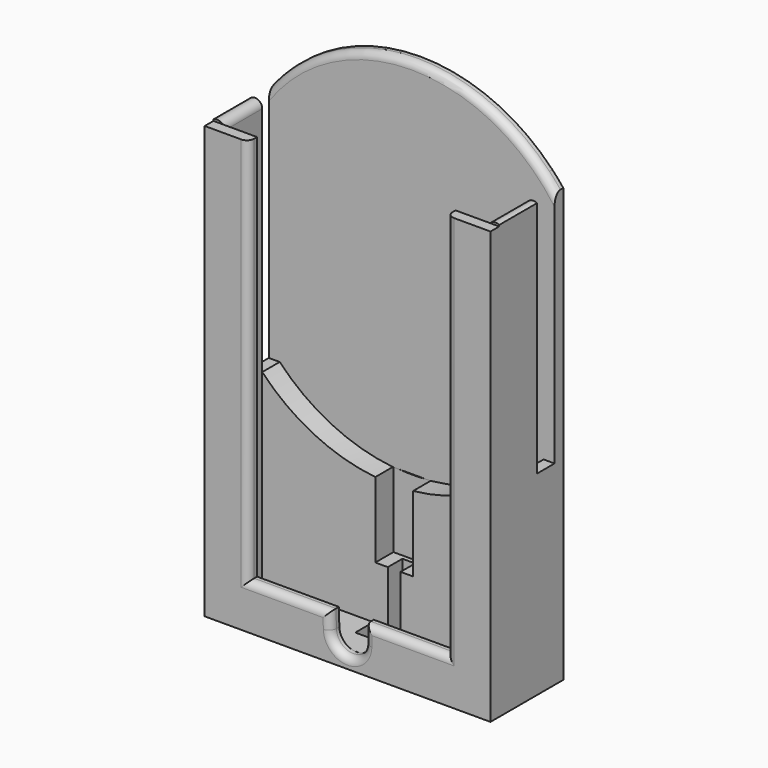
from build123d import *

# Parameters (mm, degrees)
F1_DEPTH      = 3
F2_DEPTH      = 9
F3_DEPTH      = 22
F4_DEPTH      = 22
F5_DEPTH      = 22
F6_W          = 6
F6_H          = 68.8748865698
F7_DEPTH      = 4
F8_W          = 6
F8_H          = 68.8748865698
F9_DEPTH      = 4
F10_DEPTH     = 2.8
F11_W         = 3.5
F11_H         = 14.5974665339
F12_DEPTH     = 5
F14_DEPTH     = 4
F15_DEPTH     = 4
F16_W         = 54.5
F16_H         = 12.2903782427
F17_DEPTH     = 3
F19_DEPTH     = 3
F20_T1_DEPTH  = 111.3131168485
F20_T3_DEPTH  = 27.4743105508
F20_T5_DEPTH  = 27.4558316657
F20_T7_DEPTH  = 9.7989282925
F20_T9_DEPTH  = 13
F20_T11_DEPTH = 9.7709294909
F20_T14_ANGLE = 114.906593859
F20_T16_ANGLE = 177.2719132967
F20_T21_DEPTH = 111.3131168485
F20_T25_DEPTH = 32.4558316657
F20_T32_DEPTH = 32.4743105508
F20_T36_DEPTH = 111.3131168485


# Not quite as in the source:
# - a fillet or chamfer that OpenCascade refuses, or shapes differently, is made with other operations: its cross-section is extruded or revolved along the edge and cut away or added


with BuildPart() as f1:
    # F0 (on Front) → F1 (new body)
    with BuildSketch(Plane.XZ):
        with BuildLine():
            Line((36.25, -19.4374432849), (36.25, 49.4374432849))
            ThreePointArc((36.25, 49.4374432849), (0, 65), (-36.25, 49.4374432849))
            Line((-36.25, 49.4374432849), (-36.25, -19.4374432849))
            ThreePointArc((-36.25, -19.4374432849), (-22.0820535862, -29.8595910527), (-5.1816573471, -34.7307794745))
            Line((-5.1816573471, -34.7307794745), (5.1816573471, -34.7307794745))
            ThreePointArc((5.1816573471, -34.7307794745), (22.0820535862, -29.8595910527), (36.25, -19.4374432849))
        make_face()
    extrude(amount=F1_DEPTH)

    # F0 (on Front) → F2 (join)
    with BuildSketch(Plane.XZ):
        with BuildLine():
            Line((36.25, -70), (36.25, -19.4374432849))
            ThreePointArc((36.25, -19.4374432849), (22.0820535862, -29.8595910527), (5.1816573471, -34.7307794745))
            Line((5.1816573471, -34.7307794745), (5.1816573471, -55.4025334661))
            Line((5.1816573471, -55.4025334661), (-5.1816573471, -55.4025334661))
            Line((-5.1816573471, -55.4025334661), (-5.1816573471, -34.7307794745))
            ThreePointArc((-5.1816573471, -34.7307794745), (-22.0820535862, -29.8595910527), (-36.25, -19.4374432849))
            Line((-36.25, -19.4374432849), (-36.25, -70))
            Line((-36.25, -70), (36.25, -70))
        make_face()
    extrude(amount=F2_DEPTH)

    # F0 (on Front) → F3 (join)
    with BuildSketch(Plane.XZ):
        with BuildLine():
            ThreePointArc((39.25, -15.9747881349), (37.7896810673, -17.7404948776), (36.25, -19.4374432849))
            Line((36.25, -19.4374432849), (36.25, -70))
            Line((36.25, -70), (-36.25, -70))
            Line((-36.25, -70), (-36.25, -19.4374432849))
            ThreePointArc((-36.25, -19.4374432849), (-37.7896810674, -17.7404948776), (-39.25, -15.9747881349))
            Line((-39.25, -15.9747881349), (-39.25, -73))
            Line((-39.25, -73), (39.25, -73))
            Line((39.25, -73), (39.25, -15.9747881349))
        make_face()
    extrude(amount=F3_DEPTH)

    # F0 (on Front) → F4 (join)
    with BuildSketch(Plane.XZ):
        with BuildLine():
            Line((-36.25, -19.4374432849), (-36.25, 49.4374432849))
            ThreePointArc((-36.25, 49.4374432849), (-37.7896810673, 47.7404948776), (-39.25, 45.9747881349))
            Line((-39.25, 45.9747881349), (-39.25, -15.9747881349))
            ThreePointArc((-39.25, -15.9747881349), (-37.7896810674, -17.7404948776), (-36.25, -19.4374432849))
        make_face()
    extrude(amount=F4_DEPTH)

    # F0 (on Front) → F5 (join)
    with BuildSketch(Plane.XZ):
        with BuildLine():
            ThreePointArc((39.25, 45.9747881349), (37.7896810673, 47.7404948776), (36.25, 49.4374432849))
            Line((36.25, 49.4374432849), (36.25, -19.4374432849))
            ThreePointArc((36.25, -19.4374432849), (37.7896810673, -17.7404948776), (39.25, -15.9747881349))
            Line((39.25, -15.9747881349), (39.25, 45.9747881349))
        make_face()
    extrude(amount=F5_DEPTH)

    # F6 (on face) → F7 (cut)
    with BuildSketch(Plane.YZ.offset(-36.25)):
        with Locations((-6, 15)):
            Rectangle(F6_W, F6_H)
    extrude(amount=-F7_DEPTH, mode=Mode.SUBTRACT)

    # F8 (on face) → F9 (cut)
    with BuildSketch(Plane(origin=(36.25, 0, 0), x_dir=(0, -1, 0), z_dir=(-1, 0, 0))):
        with Locations((6, 15)):
            Rectangle(F8_W, F8_H)
    extrude(amount=-F9_DEPTH, mode=Mode.SUBTRACT)

    # F0 (on Front) → F10 (join)
    with BuildSketch(Plane.XZ):
        with BuildLine():
            Line((5.1816573471, -55.4025334661), (5.1816573471, -34.7307794745))
            ThreePointArc((5.1816573471, -34.7307794745), (2.5943232525, -34.9326495077), (0, -35))
            ThreePointArc((0, -35), (-2.5943232525, -34.9326495077), (-5.1816573471, -34.7307794745))
            Line((-5.1816573471, -34.7307794745), (-5.1816573471, -55.4025334661))
            Line((-5.1816573471, -55.4025334661), (5.1816573471, -55.4025334661))
        make_face()
    extrude(amount=F10_DEPTH)

    # F11 (on face) → F12 (cut)
    with BuildSketch(Plane.XZ.offset(9)):
        with Locations((0, -62.7012667331)):
            Rectangle(F11_W, F11_H)
    extrude(amount=-F12_DEPTH, mode=Mode.SUBTRACT)

    # F13 (on face) → F14 (cut)
    with BuildSketch(Plane.XY.offset(-70)):
        Polygon((-1.75, -9), (-5.7336706668, -9), (-5.7336706668, -15.2), (5.8953360592, -15.2), (5.8953360592, -9), (1.75, -9), align=None)
    extrude(amount=-F14_DEPTH, mode=Mode.SUBTRACT)

    # F15 (cut): a face of the model
    f15_faces = [f1.faces().sort_by_distance(p)[0] for p in [
        (0, -6.5, -70),
    ]]
    extrude(f15_faces, amount=-F15_DEPTH, mode=Mode.SUBTRACT)

    # F16 (on face) → F17 (join)
    with BuildSketch(Plane.XZ.offset(22)):
        Polygon((-39.25, 45.6034950912), (-39.25, -73), (-27.25, -73), (-27.25, -60.7096217573), (-27.25, 45.6034950912), align=None)
        with Locations((0, -66.8548108786)):
            Rectangle(F16_W, F16_H)
        Polygon((27.25, -60.7096217573), (27.25, -73), (39.25, -73), (39.25, 45.6034950912), (27.25, 45.6034950912), align=None)
    extrude(amount=F17_DEPTH)

    # F18 (on face) → F19 (cut)
    with BuildSketch(Plane.XZ.offset(25)):
        with BuildLine():
            ThreePointArc((0.0047599162, -60.7096217573), (-3.3429375433, -62.1225677813), (-4.6658988973, -65.5068355016))
            ThreePointArc((-4.6658988973, -65.5068355016), (0.0184260463, -70.0542581163), (4.6760694509, -65.4795110707))
            ThreePointArc((4.6760694509, -65.4795110707), (4.6768334539, -65.4307331593), (4.6770881308, -65.3819499298))
            ThreePointArc((4.6770881308, -65.3819499298), (3.3085948781, -62.0781149802), (0.0047599162, -60.7096217573))
        make_face()
        with BuildLine():
            ThreePointArc((4.6770881308, -65.3819499298), (4.6768334539, -65.4307331593), (4.6760694509, -65.4795110707))
            Line((4.6760694509, -65.4795110707), (4.7756894492, -60.7096217573))
            Line((4.7756894492, -60.7096217573), (0.0047599162, -60.7096217573))
            ThreePointArc((0.0047599162, -60.7096217573), (3.3085948781, -62.0781149802), (4.6770881308, -65.3819499298))
        make_face()
        with BuildLine():
            Line((-4.7941683343, -60.7096217573), (-4.6658988973, -65.5068355016))
            ThreePointArc((-4.6658988973, -65.5068355016), (-3.3429375433, -62.1225677813), (0.0047599162, -60.7096217573))
            Line((0.0047599162, -60.7096217573), (-4.7941683343, -60.7096217573))
        make_face()
    extrude(amount=-F19_DEPTH, mode=Mode.SUBTRACT)

    # F20: fillet of radius 2 on 10 edges, made by hand

    # F20_s2 → F20_t1 (cut)
    with BuildSketch(Plane.XY.offset(-60.7096217573)):
        with BuildLine():
            ThreePointArc((-29.25, -25), (-27.8357864376, -24.4142135624), (-27.25, -23))
            Line((-27.25, -23), (-27.25, -25))
            Line((-27.25, -25), (-29.25, -25))
        make_face()
        with BuildLine():
            ThreePointArc((29.25, -25), (27.8357864376, -24.4142135624), (27.25, -23))
            Line((27.25, -23), (27.25, -25))
            Line((27.25, -25), (29.25, -25))
        make_face()
    extrude(amount=F20_T1_DEPTH, mode=Mode.SUBTRACT)

    # F20_s4 → F20_t3 (cut)
    with BuildSketch(Plane.YZ.offset(-0.2243105508)):
        with BuildLine():
            ThreePointArc((-25, -62.7096217573), (-24.4142135624, -61.2954081949), (-23, -60.7096217573))
            Line((-23, -60.7096217573), (-25, -60.7096217573))
            Line((-25, -60.7096217573), (-25, -62.7096217573))
        make_face()
    extrude(amount=F20_T3_DEPTH, mode=Mode.SUBTRACT)

    # F20_s6 → F20_t5 (cut)
    with BuildSketch(Plane.YZ.offset(-27.25)):
        with BuildLine():
            ThreePointArc((-25, -62.7096217573), (-24.4142135624, -61.2954081949), (-23, -60.7096217573))
            Line((-23, -60.7096217573), (-25, -60.7096217573))
            Line((-25, -60.7096217573), (-25, -62.7096217573))
        make_face()
    extrude(amount=F20_T5_DEPTH, mode=Mode.SUBTRACT)

    # F20_s8 → F20_t7 (cut)
    with BuildSketch(Plane(origin=(1.4850446734, 0, -55.5399391245), x_dir=(0, 1, 0), z_dir=(0.0267287672, 0, -0.9996427227))):
        with BuildLine():
            ThreePointArc((-25, -8.4151488306), (-24.4142135624, -7.0009352682), (-23, -6.4151488306))
            Line((-23, -6.4151488306), (-25, -6.4151488306))
            Line((-25, -6.4151488306), (-25, -8.4151488306))
        make_face()
    extrude(amount=F20_T7_DEPTH, mode=Mode.SUBTRACT)

    # F20_s10 → F20_t9 (cut)
    with BuildSketch(Plane.XZ.offset(9)):
        with BuildLine():
            ThreePointArc((39.25, 45.9747881349), (37.25, 45.9747881349), (36.25, 44.2427373273))
            Line((36.25, 44.2427373273), (36.25, 49.4374432849))
            ThreePointArc((36.25, 49.4374432849), (37.7896810673, 47.7404948776), (39.25, 45.9747881349))
        make_face()
        with BuildLine():
            ThreePointArc((-39.25, 45.9747881349), (-37.25, 45.9747881349), (-36.25, 44.2427373273))
            Line((-36.25, 44.2427373273), (-36.25, 49.4374432849))
            ThreePointArc((-36.25, 49.4374432849), (-37.7896810673, 47.7404948776), (-39.25, 45.9747881349))
        make_face()
    extrude(amount=F20_T9_DEPTH, mode=Mode.SUBTRACT)

    # F20_s12 → F20_t11 (cut)
    with BuildSketch(Plane(origin=(-1.3649163722, 0, -65.3533439927), x_dir=(0, 1, 0), z_dir=(0.0208806268, 0, 0.9997819759))):
        with BuildLine():
            ThreePointArc((-25, -8.0423031905), (-24.4142135624, -6.6280896281), (-23, -6.0423031905))
            Line((-23, -6.0423031905), (-25, -6.0423031905))
            Line((-25, -6.0423031905), (-25, -8.0423031905))
        make_face()
    extrude(amount=F20_T11_DEPTH, mode=Mode.SUBTRACT)

    # F20_s13 → F20_t14 (revolve, cut)
    with BuildSketch(Plane(origin=(6.8024666518, 0, 10.65855148), x_dir=(0, 1, 0), z_dir=(-0.537986897, 0, -0.8429532008))):
        with BuildLine():
            ThreePointArc((-1, -58.0698034549), (-2.4142135624, -57.4840170172), (-3, -56.0698034549))
            Line((-3, -56.0698034549), (-3, -58.0698034549))
            Line((-3, -58.0698034549), (-1, -58.0698034549))
        make_face()
    revolve(axis=Axis((0, -3, 15), (0, 1, 0)), revolution_arc=F20_T14_ANGLE, mode=Mode.SUBTRACT)

    # F20_s15 → F20_t16 (revolve, cut)
    with BuildSketch(Plane(origin=(1.746957946, 0, -65.3353664822), x_dir=(0, 1, 0), z_dir=(-0.0267287672, 0, 0.9996427227))):
        with BuildLine():
            ThreePointArc((-25, 8.4151488306), (-24.4142135624, 7.0009352682), (-23, 6.4151488306))
            Line((-23, 6.4151488306), (-25, 6.4151488306))
            Line((-25, 6.4151488306), (-25, 8.4151488306))
        make_face()
    revolve(axis=Axis((0.0047599583, -25, -65.3819499298), (0, -1, 0)), revolution_arc=F20_T16_ANGLE, mode=Mode.SUBTRACT)


with BuildPart() as f20_tool19:
    # F20_s20 → F20_t21 (new body)
    with BuildSketch(Plane.XY.offset(-65.7096217573)):
        with BuildLine():
            ThreePointArc((-29.25, -25), (-27.8357864376, -24.4142135624), (-27.25, -23))
            Line((-27.25, -23), (-27.25, -25))
            Line((-27.25, -25), (-29.25, -25))
        make_face()
    extrude(amount=F20_T21_DEPTH)

    split(bisect_by=Plane.XY.offset(-60.7096217573), keep=Keep.BOTTOM)


with BuildPart() as f20_tool23:
    # F20_s24 → F20_t25 (new body)
    with BuildSketch(Plane.YZ.offset(0.2058316657)):
        with BuildLine():
            ThreePointArc((-25, -62.7096217573), (-24.4142135624, -61.2954081949), (-23, -60.7096217573))
            Line((-23, -60.7096217573), (-25, -60.7096217573))
            Line((-25, -60.7096217573), (-25, -62.7096217573))
        make_face()
    extrude(amount=-F20_T25_DEPTH)

    split(bisect_by=Plane.YZ.offset(-27.25), keep=Keep.BOTTOM)


with BuildPart() as f20_tool19_1:
    add(f20_tool19.part)

    # F20_t27: intersect F20_tool23
    add(f20_tool23.part, mode=Mode.INTERSECT)


with BuildPart() as f1_1:
    add(f1.part)

    # F20_t17: cut F20_tool19
    add(f20_tool19_1.part, mode=Mode.SUBTRACT)


with BuildPart() as f20_tool30:
    # F20_s31 → F20_t32 (new body)
    with BuildSketch(Plane.YZ.offset(32.25)):
        with BuildLine():
            ThreePointArc((-25, -62.7096217573), (-24.4142135624, -61.2954081949), (-23, -60.7096217573))
            Line((-23, -60.7096217573), (-25, -60.7096217573))
            Line((-25, -60.7096217573), (-25, -62.7096217573))
        make_face()
    extrude(amount=-F20_T32_DEPTH)

    split(bisect_by=Plane.YZ.offset(27.25), keep=Keep.TOP)


with BuildPart() as f20_tool34:
    # F20_s35 → F20_t36 (new body)
    with BuildSketch(Plane.XY.offset(45.6034950912)):
        with BuildLine():
            ThreePointArc((29.25, -25), (27.8357864376, -24.4142135624), (27.25, -23))
            Line((27.25, -23), (27.25, -25))
            Line((27.25, -25), (29.25, -25))
        make_face()
    extrude(amount=-F20_T36_DEPTH)

    split(bisect_by=Plane.XY.offset(-60.7096217573), keep=Keep.BOTTOM)


with BuildPart() as f20_tool30_1:
    add(f20_tool30.part)

    # F20_t38: intersect F20_tool34
    add(f20_tool34.part, mode=Mode.INTERSECT)


with BuildPart() as f1_2:
    add(f1_1.part)

    # F20_t28: cut F20_tool30
    add(f20_tool30_1.part, mode=Mode.SUBTRACT)


solid = f1_2.part
